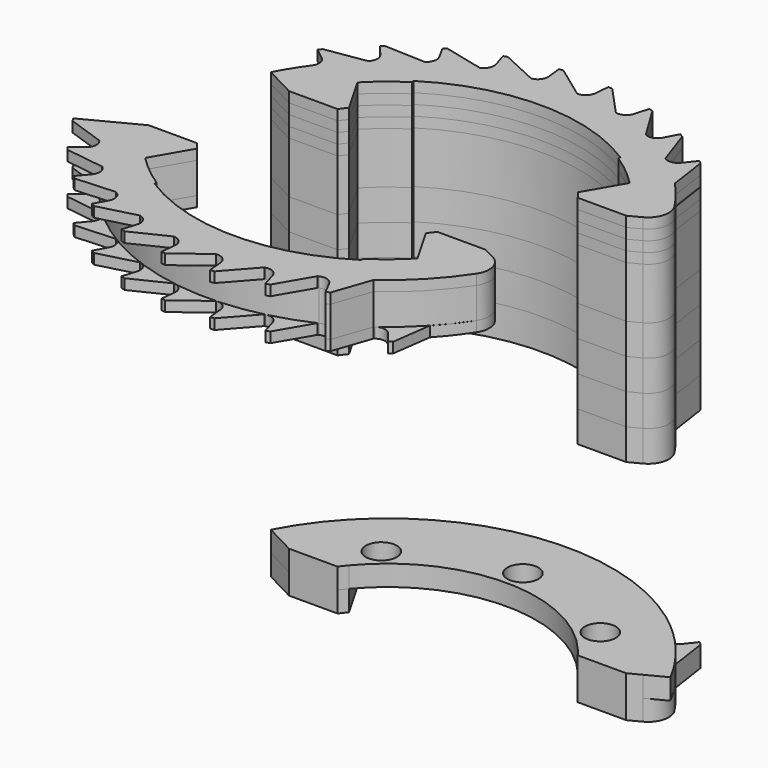
from build123d import *

# Parameters (mm, degrees)
F1_DEPTH  = 1.5
F5_DEPTH  = 0.5
F7_DEPTH  = 0.5
F9_DEPTH  = 0.5
F11_DEPTH = 0.5
F13_DEPTH = 0.5
F15_DEPTH = 0.5
F17_DEPTH = 2.5
F19_DEPTH = 1.5
F21_DEPTH = 1.5
F23_DEPTH = 1.5
F25_DEPTH = 1.5
F28_DEPTH = 1
F29_R     = 0.75
F30_DEPTH = 1


# Not quite as in the source:
# - ends of sketch curves that miss each other by under 0.0002 mm in the source are joined


with BuildPart() as f1:
    # F0 (on Top) → F1 (new body)
    with BuildSketch(Plane.XY):
        with BuildLine():
            Line((5.7645603868, -10.6404813588), (6.3916897173, -8.8292866392))
            ThreePointArc((6.3916897173, -8.8292866392), (5.5229631985, -9.3971739107), (4.6041631591, -9.8798624284))
            ThreePointArc((4.6041631591, -9.8798624284), (4.9761399678, -9.8596213915), (5.2588687206, -10.1021928204))
            Line((5.2588687206, -10.1021928204), (5.5871582201, -10.7328310815))
            Line((5.5871582201, -10.7328310815), (5.7645603868, -10.6404813588))
        make_face()
        with BuildLine():
            ThreePointArc((4.6041631591, -9.8798624284), (5.5229631985, -9.3971739107), (6.3916897173, -8.8292866392))
            ThreePointArc((6.3916897173, -8.8292866392), (7.8806152456, -7.5303322205), (9.110578105, -5.9839256841))
            ThreePointArc((9.110578105, -5.9839256841), (9.2424485693, -5.182849851), (8.7364938645, -4.5479308432))
            Line((8.7364938645, -4.5479308432), (8.1604996652, -4.2480872418))
            Line((8.1604996652, -4.2480872418), (5.813239612, -4.2480872418))
            ThreePointArc((5.813239612, -4.2480872418), (5.6789568424, -4.4259969704), (5.5392313301, -4.5996647999))
            Line((5.5392313301, -4.5996647999), (6.59, -6.4196495231))
            ThreePointArc((6.59, -6.4196495231), (5.8315097631, -7.1157215996), (5, -7.7226938305))
            Line((5, -7.7226938305), (5, -7.841555968))
            ThreePointArc((5, -7.841555968), (0, -9.3), (-5, -7.841555968))
            Line((-5, -7.841555968), (-5, -7.7226938305))
            ThreePointArc((-5, -7.7226938305), (-5.8315097631, -7.1157215996), (-6.59, -6.4196495231))
            Line((-6.59, -6.4196495231), (-5.5392313301, -4.5996647999))
            ThreePointArc((-5.5392313301, -4.5996647999), (-5.6789568424, -4.4259969704), (-5.813239612, -4.2480872418))
            Line((-5.813239612, -4.2480872418), (-8.1604996652, -4.2480872418))
            Line((-8.1604996652, -4.2480872418), (-9.6684180816, -5.0330598843))
            ThreePointArc((-9.6684180816, -5.0330598843), (-3.5049312697, -10.3211170323), (4.6041631591, -9.8798624284))
        make_face()
    extrude(amount=F1_DEPTH)


with BuildPart() as f2_1:
    # F2: copy of F1
    add(f1.part.moved(Location((0, 0, 0.5))))


with BuildPart() as f5:
    # F4 (on face) → F5 (new body)
    with BuildSketch(Plane.XY.offset(1.5)):
        with BuildLine():
            Line((5.7645603868, -10.6404813588), (6.3916897173, -8.8292866392))
            ThreePointArc((6.3916897173, -8.8292866392), (5.5229631985, -9.3971739107), (4.6041631591, -9.8798624284))
            ThreePointArc((4.6041631591, -9.8798624284), (4.9761399678, -9.8596213915), (5.2588687206, -10.1021928204))
            Line((5.2588687206, -10.1021928204), (5.5871582201, -10.7328310815))
            Line((5.5871582201, -10.7328310815), (5.7645603868, -10.6404813588))
        make_face()
        with BuildLine():
            Line((3.5779410407, -11.5606374353), (4.546366818, -9.9065911774))
            ThreePointArc((4.546366818, -9.9065911774), (3.583543325, -10.2940865179), (2.5882299124, -10.5882513155))
            ThreePointArc((2.5882299124, -10.5882513155), (2.9570081214, -10.6409682799), (3.1869809823, -10.9340364101))
            Line((3.1869809823, -10.9340364101), (3.3859310698, -11.6166032381))
            Line((3.3859310698, -11.6166032381), (3.5779410407, -11.5606374353))
        make_face()
        with BuildLine():
            Line((1.2538234269, -12.0365246984), (2.5263295915, -10.6031909723))
            ThreePointArc((2.5263295915, -10.6031909723), (1.5064098912, -10.7954031532), (0.4728324416, -10.8897396425))
            ThreePointArc((0.4728324416, -10.8897396425), (0.8242401112, -11.0133887247), (0.9926193522, -11.3456911126))
            Line((0.9926193522, -11.3456911126), (1.0545844872, -12.0539558469))
            Line((1.0545844872, -12.0539558469), (1.2538234269, -12.0365246984))
        make_face()
        with BuildLine():
            Line((-1.1184779181, -12.0498550675), (0.4092069356, -10.8923160845))
            ThreePointArc((0.4092069356, -10.8923160845), (-0.6286140299, -10.8818584994), (-1.6607357147, -10.7727413821))
            ThreePointArc((-1.6607357147, -10.7727413821), (-1.3402029842, -10.9625708173), (-1.2398880829, -11.3213372683))
            Line((-1.2398880829, -11.3213372683), (-1.3172891857, -12.0280816925))
            Line((-1.3172891857, -12.0280816925), (-1.1184779181, -12.0498550675))
        make_face()
        with BuildLine():
            Line((-3.4477967839, -11.600116264), (-1.7236413133, -10.762855598))
            ThreePointArc((-1.7236413133, -10.762855598), (-2.7394806663, -10.5501301262), (-3.7304827288, -10.2417527118))
            ThreePointArc((-3.7304827288, -10.2417527118), (-3.4531428306, -10.4904674612), (-3.4247473144, -10.8619107818))
            Line((-3.4247473144, -10.8619107818), (-3.638540174, -11.5399751041))
            Line((-3.638540174, -11.5399751041), (-3.4477967839, -11.600116264))
        make_face()
        with BuildLine():
            Line((-5.6446187528, -10.7045914978), (-3.7902509932, -10.2197846068))
            ThreePointArc((-3.7902509932, -10.2197846068), (-4.7450705971, -9.8129661687), (-5.6568693838, -9.3171792284))
            ThreePointArc((-5.6568693838, -9.3171792284), (-5.4333803345, -9.6152213237), (-5.4779954272, -9.9850671555))
            Line((-5.4779954272, -9.9850671555), (-5.8199641039, -10.6083937441))
            Line((-5.8199641039, -10.6083937441), (-5.6446187528, -10.7045914978))
        make_face()
        with BuildLine():
            Line((-7.6245211886, -9.3976952837), (-5.711203453, -9.2839730244))
            ThreePointArc((-5.711203453, -9.2839730244), (-6.5683101259, -8.6986954246), (-7.3658657208, -8.0345517724))
            ThreePointArc((-7.3658657208, -8.0345517724), (-7.2048160792, -8.3704676231), (-7.3207272478, -8.724502998))
            Line((-7.3207272478, -8.724502998), (-7.7777300772, -9.2691377617))
            Line((-7.7777300772, -9.2691377617), (-7.6245211886, -9.3976952837))
        make_face()
        with BuildLine():
            Line((-9.311417551, -7.72965091), (-7.4126775671, -7.9913835652))
            ThreePointArc((-7.4126775671, -7.9913835652), (-8.1391331801, -7.2501386936), (-8.7917959689, -6.4431609976))
            ThreePointArc((-8.7917959689, -6.4431609976), (-8.6993747825, -6.8040415458), (-8.8821276259, -7.1286610831))
            Line((-8.8821276259, -7.1286610831), (-9.4366022454, -7.5736740134))
            Line((-9.4366022454, -7.5736740134), (-9.311417551, -7.72965091))
        make_face()
        with BuildLine():
            ThreePointArc((-8.8292866392, -6.3916897173), (-9.2737661573, -5.7277623256), (-9.6684180816, -5.0330598843))
            Line((-9.6684180816, -5.0330598843), (-10.1021928204, -5.2588687206))
            Line((-10.1021928204, -5.2588687206), (-10.7328310815, -5.5871582201))
            Line((-10.7328310815, -5.5871582201), (-10.6404813588, -5.7645603868))
            Line((-10.6404813588, -5.7645603868), (-8.8292866392, -6.3916897173))
        make_face()
        with BuildLine():
            ThreePointArc((4.6041631591, -9.8798624284), (5.5229631985, -9.3971739107), (6.3916897173, -8.8292866392))
            ThreePointArc((6.3916897173, -8.8292866392), (7.8806152456, -7.5303322205), (9.110578105, -5.9839256841))
            ThreePointArc((9.110578105, -5.9839256841), (9.2424485693, -5.182849851), (8.7364938645, -4.5479308432))
            Line((8.7364938645, -4.5479308432), (8.1604996652, -4.2480872418))
            Line((8.1604996652, -4.2480872418), (5.813239612, -4.2480872418))
            ThreePointArc((5.813239612, -4.2480872418), (5.6789568424, -4.4259969704), (5.5392313301, -4.5996647999))
            Line((5.5392313301, -4.5996647999), (6.59, -6.4196495231))
            ThreePointArc((6.59, -6.4196495231), (5.8315097631, -7.1157215996), (5, -7.7226938305))
            Line((5, -7.7226938305), (5, -7.841555968))
            ThreePointArc((5, -7.841555968), (0, -9.3), (-5, -7.841555968))
            Line((-5, -7.841555968), (-5, -7.7226938305))
            ThreePointArc((-5, -7.7226938305), (-5.8315097631, -7.1157215996), (-6.59, -6.4196495231))
            Line((-6.59, -6.4196495231), (-5.5392313301, -4.5996647999))
            ThreePointArc((-5.5392313301, -4.5996647999), (-5.6789568424, -4.4259969704), (-5.813239612, -4.2480872418))
            Line((-5.813239612, -4.2480872418), (-8.1604996652, -4.2480872418))
            Line((-8.1604996652, -4.2480872418), (-9.6684180816, -5.0330598843))
            ThreePointArc((-9.6684180816, -5.0330598843), (-9.2737661573, -5.7277623256), (-8.8292866392, -6.3916897173))
            ThreePointArc((-8.8292866392, -6.3916897173), (-8.810578891, -6.417452735), (-8.7917959689, -6.4431609976))
            ThreePointArc((-8.7917959689, -6.4431609976), (-8.1391331801, -7.2501386936), (-7.4126775671, -7.9913835652))
            ThreePointArc((-7.4126775671, -7.9913835652), (-7.3893031675, -8.0130018532), (-7.3658657208, -8.0345517724))
            ThreePointArc((-7.3658657208, -8.0345517724), (-6.5683101259, -8.6986954246), (-5.711203453, -9.2839730244))
            ThreePointArc((-5.711203453, -9.2839730244), (-5.6840606672, -9.3006158039), (-5.6568693838, -9.3171792284))
            ThreePointArc((-5.6568693838, -9.3171792284), (-4.7450705971, -9.8129661687), (-3.7902509932, -10.2197846068))
            ThreePointArc((-3.7902509932, -10.2197846068), (-3.7603829032, -10.230812305), (-3.7304827288, -10.2417527118))
            ThreePointArc((-3.7304827288, -10.2417527118), (-2.7394806663, -10.5501301262), (-1.7236413133, -10.762855598))
            ThreePointArc((-1.7236413133, -10.762855598), (-1.6921957331, -10.7678444269), (-1.6607357147, -10.7727413821))
            ThreePointArc((-1.6607357147, -10.7727413821), (-0.6286140299, -10.8818584994), (0.4092069356, -10.8923160845))
            ThreePointArc((0.4092069356, -10.8923160845), (0.4410215701, -10.891074326), (0.4728324416, -10.8897396425))
            ThreePointArc((0.4728324416, -10.8897396425), (1.5064098912, -10.7954031532), (2.5263295915, -10.6031909723))
            ThreePointArc((2.5263295915, -10.6031909723), (2.5572906616, -10.5957663466), (2.5882299124, -10.5882513155))
            ThreePointArc((2.5882299124, -10.5882513155), (3.583543325, -10.2940865179), (4.546366818, -9.9065911774))
            ThreePointArc((4.546366818, -9.9065911774), (4.5752845072, -9.8932690087), (4.6041631591, -9.8798624284))
        make_face()
    extrude(amount=F5_DEPTH)


with BuildPart() as f7:
    # F6 (on Top) → F7 (new body)
    with BuildSketch(Plane.XY):
        with BuildLine():
            Line((5.7645603868, -10.6404813588), (6.3916897173, -8.8292866392))
            ThreePointArc((6.3916897173, -8.8292866392), (5.5229631985, -9.3971739107), (4.6041631591, -9.8798624284))
            ThreePointArc((4.6041631591, -9.8798624284), (4.9761399678, -9.8596213915), (5.2588687206, -10.1021928204))
            Line((5.2588687206, -10.1021928204), (5.5871582201, -10.7328310815))
            Line((5.5871582201, -10.7328310815), (5.7645603868, -10.6404813588))
        make_face()
        with BuildLine():
            ThreePointArc((4.6041631591, -9.8798624284), (5.5229631985, -9.3971739107), (6.3916897173, -8.8292866392))
            ThreePointArc((6.3916897173, -8.8292866392), (6.417452735, -8.810578891), (6.4431609976, -8.7917959689))
            ThreePointArc((6.4431609976, -8.7917959689), (7.2501386936, -8.1391331801), (7.9913835652, -7.4126775671))
            ThreePointArc((7.9913835652, -7.4126775671), (8.5807695592, -6.7216362422), (9.110578105, -5.9839256841))
            ThreePointArc((9.110578105, -5.9839256841), (9.2424485693, -5.182849851), (8.7364938645, -4.5479308432))
            Line((8.7364938645, -4.5479308432), (8.1604996652, -4.2480872418))
            Line((8.1604996652, -4.2480872418), (5.813239612, -4.2480872418))
            ThreePointArc((5.813239612, -4.2480872418), (5.6789568424, -4.4259969704), (5.5392313301, -4.5996647999))
            Line((5.5392313301, -4.5996647999), (6.59, -6.4196495231))
            ThreePointArc((6.59, -6.4196495231), (5.8315097631, -7.1157215996), (5, -7.7226938305))
            Line((5, -7.7226938305), (5, -7.841555968))
            ThreePointArc((5, -7.841555968), (0, -9.3), (-5, -7.841555968))
            Line((-5, -7.841555968), (-5, -7.7226938305))
            ThreePointArc((-5, -7.7226938305), (-5.8315097631, -7.1157215996), (-6.59, -6.4196495231))
            Line((-6.59, -6.4196495231), (-5.5392313301, -4.5996647999))
            ThreePointArc((-5.5392313301, -4.5996647999), (-5.6789568424, -4.4259969704), (-5.813239612, -4.2480872418))
            Line((-5.813239612, -4.2480872418), (-8.1604996652, -4.2480872418))
            Line((-8.1604996652, -4.2480872418), (-9.6684180816, -5.0330598843))
            ThreePointArc((-9.6684180816, -5.0330598843), (-9.2737661573, -5.7277623256), (-8.8292866392, -6.3916897173))
            ThreePointArc((-8.8292866392, -6.3916897173), (-8.810578891, -6.417452735), (-8.7917959689, -6.4431609976))
            ThreePointArc((-8.7917959689, -6.4431609976), (-8.1391331801, -7.2501386936), (-7.4126775671, -7.9913835652))
            ThreePointArc((-7.4126775671, -7.9913835652), (-7.3893031675, -8.0130018532), (-7.3658657208, -8.0345517724))
            ThreePointArc((-7.3658657208, -8.0345517724), (-6.5683101259, -8.6986954246), (-5.711203453, -9.2839730244))
            ThreePointArc((-5.711203453, -9.2839730244), (-5.6840606672, -9.3006158039), (-5.6568693838, -9.3171792284))
            ThreePointArc((-5.6568693838, -9.3171792284), (-4.7450705971, -9.8129661687), (-3.7902509932, -10.2197846068))
            ThreePointArc((-3.7902509932, -10.2197846068), (-3.7603829032, -10.230812305), (-3.7304827288, -10.2417527118))
            ThreePointArc((-3.7304827288, -10.2417527118), (-2.7394806663, -10.5501301262), (-1.7236413133, -10.762855598))
            ThreePointArc((-1.7236413133, -10.762855598), (-1.6921957331, -10.7678444269), (-1.6607357147, -10.7727413821))
            ThreePointArc((-1.6607357147, -10.7727413821), (-0.6286140299, -10.8818584994), (0.4092069356, -10.8923160845))
            ThreePointArc((0.4092069356, -10.8923160845), (0.4410215701, -10.891074326), (0.4728324416, -10.8897396425))
            ThreePointArc((0.4728324416, -10.8897396425), (1.5064098912, -10.7954031532), (2.5263295915, -10.6031909723))
            ThreePointArc((2.5263295915, -10.6031909723), (2.5572906616, -10.5957663466), (2.5882299124, -10.5882513155))
            ThreePointArc((2.5882299124, -10.5882513155), (3.583543325, -10.2940865179), (4.546366818, -9.9065911774))
            ThreePointArc((4.546366818, -9.9065911774), (4.5752845072, -9.8932690087), (4.6041631591, -9.8798624284))
        make_face()
        with BuildLine():
            ThreePointArc((7.9913835652, -7.4126775671), (7.2501386936, -8.1391331801), (6.4431609976, -8.7917959689))
            ThreePointArc((6.4431609976, -8.7917959689), (6.8040415458, -8.6993747825), (7.1286610831, -8.8821276259))
            Line((7.1286610831, -8.8821276259), (7.5736740134, -9.4366022454))
            Line((7.5736740134, -9.4366022454), (7.72965091, -9.311417551))
            Line((7.72965091, -9.311417551), (7.9913835652, -7.4126775671))
        make_face()
        with BuildLine():
            Line((3.5779410407, -11.5606374353), (4.546366818, -9.9065911774))
            ThreePointArc((4.546366818, -9.9065911774), (3.583543325, -10.2940865179), (2.5882299124, -10.5882513155))
            ThreePointArc((2.5882299124, -10.5882513155), (2.9570081214, -10.6409682799), (3.1869809823, -10.9340364101))
            Line((3.1869809823, -10.9340364101), (3.3859310698, -11.6166032381))
            Line((3.3859310698, -11.6166032381), (3.5779410407, -11.5606374353))
        make_face()
        with BuildLine():
            Line((1.2538234269, -12.0365246984), (2.5263295915, -10.6031909723))
            ThreePointArc((2.5263295915, -10.6031909723), (1.5064098912, -10.7954031532), (0.4728324416, -10.8897396425))
            ThreePointArc((0.4728324416, -10.8897396425), (0.8242401112, -11.0133887247), (0.9926193522, -11.3456911126))
            Line((0.9926193522, -11.3456911126), (1.0545844872, -12.0539558469))
            Line((1.0545844872, -12.0539558469), (1.2538234269, -12.0365246984))
        make_face()
        with BuildLine():
            Line((-1.1184779181, -12.0498550675), (0.4092069356, -10.8923160845))
            ThreePointArc((0.4092069356, -10.8923160845), (-0.6286140299, -10.8818584994), (-1.6607357147, -10.7727413821))
            ThreePointArc((-1.6607357147, -10.7727413821), (-1.3402029842, -10.9625708173), (-1.2398880829, -11.3213372683))
            Line((-1.2398880829, -11.3213372683), (-1.3172891857, -12.0280816925))
            Line((-1.3172891857, -12.0280816925), (-1.1184779181, -12.0498550675))
        make_face()
        with BuildLine():
            Line((-3.4477967839, -11.600116264), (-1.7236413133, -10.762855598))
            ThreePointArc((-1.7236413133, -10.762855598), (-2.7394806663, -10.5501301262), (-3.7304827288, -10.2417527118))
            ThreePointArc((-3.7304827288, -10.2417527118), (-3.4531428306, -10.4904674612), (-3.4247473144, -10.8619107818))
            Line((-3.4247473144, -10.8619107818), (-3.638540174, -11.5399751041))
            Line((-3.638540174, -11.5399751041), (-3.4477967839, -11.600116264))
        make_face()
        with BuildLine():
            Line((-5.6446187528, -10.7045914978), (-3.7902509932, -10.2197846068))
            ThreePointArc((-3.7902509932, -10.2197846068), (-4.7450705971, -9.8129661687), (-5.6568693838, -9.3171792284))
            ThreePointArc((-5.6568693838, -9.3171792284), (-5.4333803345, -9.6152213237), (-5.4779954272, -9.9850671555))
            Line((-5.4779954272, -9.9850671555), (-5.8199641039, -10.6083937441))
            Line((-5.8199641039, -10.6083937441), (-5.6446187528, -10.7045914978))
        make_face()
        with BuildLine():
            Line((-7.6245211886, -9.3976952837), (-5.711203453, -9.2839730244))
            ThreePointArc((-5.711203453, -9.2839730244), (-6.5683101259, -8.6986954246), (-7.3658657208, -8.0345517724))
            ThreePointArc((-7.3658657208, -8.0345517724), (-7.2048160792, -8.3704676231), (-7.3207272478, -8.724502998))
            Line((-7.3207272478, -8.724502998), (-7.7777300772, -9.2691377617))
            Line((-7.7777300772, -9.2691377617), (-7.6245211886, -9.3976952837))
        make_face()
        with BuildLine():
            Line((-9.311417551, -7.72965091), (-7.4126775671, -7.9913835652))
            ThreePointArc((-7.4126775671, -7.9913835652), (-8.1391331801, -7.2501386936), (-8.7917959689, -6.4431609976))
            ThreePointArc((-8.7917959689, -6.4431609976), (-8.6993747825, -6.8040415458), (-8.8821276259, -7.1286610831))
            Line((-8.8821276259, -7.1286610831), (-9.4366022454, -7.5736740134))
            Line((-9.4366022454, -7.5736740134), (-9.311417551, -7.72965091))
        make_face()
        with BuildLine():
            Line((-10.6404813588, -5.7645603868), (-8.8292866392, -6.3916897173))
            ThreePointArc((-8.8292866392, -6.3916897173), (-9.2737661573, -5.7277623256), (-9.6684180816, -5.0330598843))
            Line((-9.6684180816, -5.0330598843), (-10.1021928204, -5.2588687206))
            Line((-10.1021928204, -5.2588687206), (-10.7328310815, -5.5871582201))
            Line((-10.7328310815, -5.5871582201), (-10.6404813588, -5.7645603868))
        make_face()
    extrude(amount=-F7_DEPTH)


with BuildPart() as f9:
    # F8 (on face) → F9 (new body)
    with BuildSketch(Plane(origin=(0, 0, -0.5), x_dir=(1, 0, 0), z_dir=(0, 0, -1))):
        with BuildLine():
            Line((5.7645603868, -10.6404813588), (6.3916897173, -8.8292866392))
            ThreePointArc((6.3916897173, -8.8292866392), (5.5229631985, -9.3971739107), (4.6041631591, -9.8798624284))
            ThreePointArc((4.6041631591, -9.8798624284), (4.9761399678, -9.8596213915), (5.2588687206, -10.1021928204))
            Line((5.2588687206, -10.1021928204), (5.5871582201, -10.7328310815))
            Line((5.5871582201, -10.7328310815), (5.7645603868, -10.6404813588))
        make_face()
        with BuildLine():
            Line((3.5779410407, -11.5606374353), (4.6041631591, -9.8798624284))
            ThreePointArc((4.6041631591, -9.8798624284), (3.613596993, -10.2835750968), (2.5882299124, -10.5882513155))
            ThreePointArc((2.5882299124, -10.5882513155), (2.9570081214, -10.6409682799), (3.1869809823, -10.9340364101))
            Line((3.1869809823, -10.9340364101), (3.3859310698, -11.6166032381))
            Line((3.3859310698, -11.6166032381), (3.5779410407, -11.5606374353))
        make_face()
        with BuildLine():
            Line((1.2538234269, -12.0365246984), (2.5882299124, -10.5882513155))
            ThreePointArc((2.5882299124, -10.5882513155), (1.5379367629, -10.7909568859), (0.4728324416, -10.8897396425))
            ThreePointArc((0.4728324416, -10.8897396425), (0.8242401112, -11.0133887247), (0.9926193522, -11.3456911126))
            Line((0.9926193522, -11.3456911126), (1.0545844872, -12.0539558469))
            Line((1.0545844872, -12.0539558469), (1.2538234269, -12.0365246984))
        make_face()
        with BuildLine():
            Line((-1.1184779181, -12.0498550675), (0.4728324416, -10.8897396425))
            ThreePointArc((0.4728324416, -10.8897396425), (-0.5968255145, -10.8836482535), (-1.6607357147, -10.7727413821))
            ThreePointArc((-1.6607357147, -10.7727413821), (-1.3402029842, -10.9625708173), (-1.2398880829, -11.3213372683))
            Line((-1.2398880829, -11.3213372683), (-1.3172891857, -12.0280816925))
            Line((-1.3172891857, -12.0280816925), (-1.1184779181, -12.0498550675))
        make_face()
        with BuildLine():
            Line((-3.4477967839, -11.600116264), (-1.6607357147, -10.7727413821))
            ThreePointArc((-1.6607357147, -10.7727413821), (-2.7086521221, -10.5580871223), (-3.7304827288, -10.2417527118))
            ThreePointArc((-3.7304827288, -10.2417527118), (-3.4531428306, -10.4904674612), (-3.4247473144, -10.8619107818))
            Line((-3.4247473144, -10.8619107818), (-3.638540174, -11.5399751041))
            Line((-3.638540174, -11.5399751041), (-3.4477967839, -11.600116264))
        make_face()
        with BuildLine():
            Line((-5.6446187528, -10.7045914978), (-3.7304827288, -10.2417527118))
            ThreePointArc((-3.7304827288, -10.2417527118), (-4.7163867476, -9.826784624), (-5.6568693838, -9.3171792284))
            ThreePointArc((-5.6568693838, -9.3171792284), (-5.4333803345, -9.6152213237), (-5.4779954272, -9.9850671555))
            Line((-5.4779954272, -9.9850671555), (-5.8199641039, -10.6083937441))
            Line((-5.8199641039, -10.6083937441), (-5.6446187528, -10.7045914978))
        make_face()
        with BuildLine():
            Line((-7.6245211886, -9.3976952837), (-5.6568693838, -9.3171792284))
            ThreePointArc((-5.6568693838, -9.3171792284), (-6.5428732754, -8.7178443036), (-7.3658657208, -8.0345517724))
            ThreePointArc((-7.3658657208, -8.0345517724), (-7.2048160792, -8.3704676231), (-7.3207272478, -8.724502998))
            Line((-7.3207272478, -8.724502998), (-7.7777300772, -9.2691377617))
            Line((-7.7777300772, -9.2691377617), (-7.6245211886, -9.3976952837))
        make_face()
        with BuildLine():
            Line((-9.311417551, -7.72965091), (-7.3658657208, -8.0345517724))
            ThreePointArc((-7.3658657208, -8.0345517724), (-8.1179208526, -7.2738821156), (-8.7917959689, -6.4431609976))
            ThreePointArc((-8.7917959689, -6.4431609976), (-8.6993747825, -6.8040415458), (-8.8821276259, -7.1286610831))
            Line((-8.8821276259, -7.1286610831), (-9.4366022454, -7.5736740134))
            Line((-9.4366022454, -7.5736740134), (-9.311417551, -7.72965091))
        make_face()
        with BuildLine():
            ThreePointArc((7.9451671881, -7.4621925969), (7.2009445916, -8.1826888606), (6.3916897173, -8.8292866392))
            ThreePointArc((6.3916897173, -8.8292866392), (6.7529700924, -8.7384409661), (7.0767891323, -8.9226084852))
            Line((7.0767891323, -8.9226084852), (7.5193784822, -9.4790195556))
            Line((7.5193784822, -9.4790195556), (7.6759001136, -9.3545166283))
            Line((7.6759001136, -9.3545166283), (7.9451671881, -7.4621925969))
        make_face()
        with BuildLine():
            ThreePointArc((4.6041631591, -9.8798624284), (5.5229631985, -9.3971739107), (6.3916897173, -8.8292866392))
            ThreePointArc((6.3916897173, -8.8292866392), (7.2009445916, -8.1826888606), (7.9451671881, -7.4621925969))
            ThreePointArc((7.9451671881, -7.4621925969), (8.5598440489, -6.7482642108), (9.110578105, -5.9839256841))
            ThreePointArc((9.110578105, -5.9839256841), (9.2424485693, -5.182849851), (8.7364938645, -4.5479308432))
            Line((8.7364938645, -4.5479308432), (8.1604996652, -4.2480872418))
            Line((8.1604996652, -4.2480872418), (5.813239612, -4.2480872418))
            ThreePointArc((5.813239612, -4.2480872418), (5.6789568424, -4.4259969704), (5.5392313301, -4.5996647999))
            Line((5.5392313301, -4.5996647999), (6.59, -6.4196495231))
            ThreePointArc((6.59, -6.4196495231), (5.8315097631, -7.1157215996), (5, -7.7226938305))
            Line((5, -7.7226938305), (5, -7.841555968))
            ThreePointArc((5, -7.841555968), (0, -9.3), (-5, -7.841555968))
            Line((-5, -7.841555968), (-5, -7.7226938305))
            ThreePointArc((-5, -7.7226938305), (-5.8315097631, -7.1157215996), (-6.59, -6.4196495231))
            Line((-6.59, -6.4196495231), (-5.5392313301, -4.5996647999))
            ThreePointArc((-5.5392313301, -4.5996647999), (-5.6789568424, -4.4259969704), (-5.813239612, -4.2480872418))
            Line((-5.813239612, -4.2480872418), (-8.1604996652, -4.2480872418))
            Line((-8.1604996652, -4.2480872418), (-9.6684180816, -5.0330598843))
            ThreePointArc((-9.6684180816, -5.0330598843), (-9.2569958402, -5.7548264974), (-8.7917959689, -6.4431609976))
            ThreePointArc((-8.7917959689, -6.4431609976), (-8.1179208526, -7.2738821156), (-7.3658657208, -8.0345517724))
            ThreePointArc((-7.3658657208, -8.0345517724), (-6.5428732754, -8.7178443036), (-5.6568693838, -9.3171792284))
            ThreePointArc((-5.6568693838, -9.3171792284), (-4.7163867476, -9.826784624), (-3.7304827288, -10.2417527118))
            ThreePointArc((-3.7304827288, -10.2417527118), (-2.7086521221, -10.5580871223), (-1.6607357147, -10.7727413821))
            ThreePointArc((-1.6607357147, -10.7727413821), (-0.5968255145, -10.8836482535), (0.4728324416, -10.8897396425))
            ThreePointArc((0.4728324416, -10.8897396425), (1.5379367629, -10.7909568859), (2.5882299124, -10.5882513155))
            ThreePointArc((2.5882299124, -10.5882513155), (3.613596993, -10.2835750968), (4.6041631591, -9.8798624284))
        make_face()
    extrude(amount=-F9_DEPTH)


with BuildPart() as f11:
    # F10 (on face) → F11 (new body)
    with BuildSketch(Plane(origin=(0, 0, -0.5), x_dir=(1, 0, 0), z_dir=(0, 0, -1))):
        with BuildLine():
            Line((5.7645603868, -10.6404813588), (6.3916897173, -8.8292866392))
            ThreePointArc((6.3916897173, -8.8292866392), (5.5229631985, -9.3971739107), (4.6041631591, -9.8798624284))
            ThreePointArc((4.6041631591, -9.8798624284), (4.9761399678, -9.8596213915), (5.2588687206, -10.1021928204))
            Line((5.2588687206, -10.1021928204), (5.5871582201, -10.7328310815))
            Line((5.5871582201, -10.7328310815), (5.7645603868, -10.6404813588))
        make_face()
        with BuildLine():
            ThreePointArc((4.6041631591, -9.8798624284), (5.5229631985, -9.3971739107), (6.3916897173, -8.8292866392))
            ThreePointArc((6.3916897173, -8.8292866392), (7.2009445916, -8.1826888606), (7.9451671881, -7.4621925969))
            ThreePointArc((7.9451671881, -7.4621925969), (8.5598440489, -6.7482642108), (9.110578105, -5.9839256841))
            ThreePointArc((9.110578105, -5.9839256841), (9.2424485693, -5.182849851), (8.7364938645, -4.5479308432))
            Line((8.7364938645, -4.5479308432), (8.1604996652, -4.2480872418))
            Line((8.1604996652, -4.2480872418), (5.813239612, -4.2480872418))
            ThreePointArc((5.813239612, -4.2480872418), (5.6789568424, -4.4259969704), (5.5392313301, -4.5996647999))
            Line((5.5392313301, -4.5996647999), (6.59, -6.4196495231))
            ThreePointArc((6.59, -6.4196495231), (5.8315097631, -7.1157215996), (5, -7.7226938305))
            Line((5, -7.7226938305), (5, -7.841555968))
            ThreePointArc((5, -7.841555968), (0, -9.3), (-5, -7.841555968))
            Line((-5, -7.841555968), (-5, -7.7226938305))
            ThreePointArc((-5, -7.7226938305), (-5.8315097631, -7.1157215996), (-6.59, -6.4196495231))
            Line((-6.59, -6.4196495231), (-5.5392313301, -4.5996647999))
            ThreePointArc((-5.5392313301, -4.5996647999), (-5.6789568424, -4.4259969704), (-5.813239612, -4.2480872418))
            Line((-5.813239612, -4.2480872418), (-8.1604996652, -4.2480872418))
            Line((-8.1604996652, -4.2480872418), (-9.6684180816, -5.0330598843))
            ThreePointArc((-9.6684180816, -5.0330598843), (-8.6483492387, -6.6344596951), (-7.3658657208, -8.0345517724))
            ThreePointArc((-7.3658657208, -8.0345517724), (-6.5428732754, -8.7178443036), (-5.6568693838, -9.3171792284))
            ThreePointArc((-5.6568693838, -9.3171792284), (-4.7163867476, -9.826784624), (-3.7304827288, -10.2417527118))
            ThreePointArc((-3.7304827288, -10.2417527118), (-2.7086521221, -10.5580871223), (-1.6607357147, -10.7727413821))
            ThreePointArc((-1.6607357147, -10.7727413821), (-0.5968255145, -10.8836482535), (0.4728324416, -10.8897396425))
            ThreePointArc((0.4728324416, -10.8897396425), (1.5379367629, -10.7909568859), (2.5882299124, -10.5882513155))
            ThreePointArc((2.5882299124, -10.5882513155), (3.613596993, -10.2835750968), (4.6041631591, -9.8798624284))
        make_face()
        with BuildLine():
            ThreePointArc((7.9451671881, -7.4621925969), (7.2009445916, -8.1826888606), (6.3916897173, -8.8292866392))
            ThreePointArc((6.3916897173, -8.8292866392), (6.7529700924, -8.7384409661), (7.0767891323, -8.9226084852))
            Line((7.0767891323, -8.9226084852), (7.5193784822, -9.4790195556))
            Line((7.5193784822, -9.4790195556), (7.6759001136, -9.3545166283))
            Line((7.6759001136, -9.3545166283), (7.9451671881, -7.4621925969))
        make_face()
        with BuildLine():
            Line((3.5779410407, -11.5606374353), (4.6041631591, -9.8798624284))
            ThreePointArc((4.6041631591, -9.8798624284), (3.613596993, -10.2835750968), (2.5882299124, -10.5882513155))
            ThreePointArc((2.5882299124, -10.5882513155), (2.9570081214, -10.6409682799), (3.1869809823, -10.9340364101))
            Line((3.1869809823, -10.9340364101), (3.3859310698, -11.6166032381))
            Line((3.3859310698, -11.6166032381), (3.5779410407, -11.5606374353))
        make_face()
        with BuildLine():
            Line((1.2538234269, -12.0365246984), (2.5882299124, -10.5882513155))
            ThreePointArc((2.5882299124, -10.5882513155), (1.5379367629, -10.7909568859), (0.4728324416, -10.8897396425))
            ThreePointArc((0.4728324416, -10.8897396425), (0.8242401112, -11.0133887247), (0.9926193522, -11.3456911126))
            Line((0.9926193522, -11.3456911126), (1.0545844872, -12.0539558469))
            Line((1.0545844872, -12.0539558469), (1.2538234269, -12.0365246984))
        make_face()
        with BuildLine():
            Line((-1.1184779181, -12.0498550675), (0.4728324416, -10.8897396425))
            ThreePointArc((0.4728324416, -10.8897396425), (-0.5968255145, -10.8836482535), (-1.6607357147, -10.7727413821))
            ThreePointArc((-1.6607357147, -10.7727413821), (-1.3402029842, -10.9625708173), (-1.2398880829, -11.3213372683))
            Line((-1.2398880829, -11.3213372683), (-1.3172891857, -12.0280816925))
            Line((-1.3172891857, -12.0280816925), (-1.1184779181, -12.0498550675))
        make_face()
        with BuildLine():
            Line((-3.4477967839, -11.600116264), (-1.6607357147, -10.7727413821))
            ThreePointArc((-1.6607357147, -10.7727413821), (-2.7086521221, -10.5580871223), (-3.7304827288, -10.2417527118))
            ThreePointArc((-3.7304827288, -10.2417527118), (-3.4531428306, -10.4904674612), (-3.4247473144, -10.8619107818))
            Line((-3.4247473144, -10.8619107818), (-3.638540174, -11.5399751041))
            Line((-3.638540174, -11.5399751041), (-3.4477967839, -11.600116264))
        make_face()
        with BuildLine():
            Line((-5.6446187528, -10.7045914978), (-3.7304827288, -10.2417527118))
            ThreePointArc((-3.7304827288, -10.2417527118), (-4.7163867476, -9.826784624), (-5.6568693838, -9.3171792284))
            ThreePointArc((-5.6568693838, -9.3171792284), (-5.4333803345, -9.6152213237), (-5.4779954272, -9.9850671555))
            Line((-5.4779954272, -9.9850671555), (-5.8199641039, -10.6083937441))
            Line((-5.8199641039, -10.6083937441), (-5.6446187528, -10.7045914978))
        make_face()
        with BuildLine():
            Line((-7.6245211886, -9.3976952837), (-5.6568693838, -9.3171792284))
            ThreePointArc((-5.6568693838, -9.3171792284), (-6.5428732754, -8.7178443036), (-7.3658657208, -8.0345517724))
            ThreePointArc((-7.3658657208, -8.0345517724), (-7.2048160792, -8.3704676231), (-7.3207272478, -8.724502998))
            Line((-7.3207272478, -8.724502998), (-7.7777300772, -9.2691377617))
            Line((-7.7777300772, -9.2691377617), (-7.6245211886, -9.3976952837))
        make_face()
    extrude(amount=F11_DEPTH)


with BuildPart() as f13:
    # F12 (on face) → F13 (new body)
    with BuildSketch(Plane(origin=(0, 0, -1), x_dir=(1, 0, 0), z_dir=(0, 0, -1))):
        with BuildLine():
            ThreePointArc((9.1100288204, -5.984761891), (9.1103035022, -5.9843437482), (9.1105781649, -5.9839255929))
            ThreePointArc((9.1105781649, -5.9839255929), (9.2424486233, -5.1828497668), (8.7364939254, -4.5479307637))
            Line((8.7364939254, -4.5479307637), (8.160499713, -4.2480871501))
            Line((8.160499713, -4.2480871501), (5.813239679, -4.2480871501))
            ThreePointArc((5.813239679, -4.2480871501), (5.6789569122, -4.4259968809), (5.5392314026, -4.5996647126))
            Line((5.5392314026, -4.5996647126), (6.59, -6.4196495231))
            ThreePointArc((6.59, -6.4196495231), (5.8315097631, -7.1157215996), (5, -7.7226938305))
            Line((5, -7.7226938305), (5, -7.841555968))
            ThreePointArc((5, -7.841555968), (0, -9.3), (-5, -7.841555968))
            Line((-5, -7.841555968), (-5, -7.7226938305))
            ThreePointArc((-5, -7.7226938305), (-5.8315097631, -7.1157215996), (-6.59, -6.4196495231))
            Line((-6.59, -6.4196495231), (-5.5392312576, -4.5996648872))
            ThreePointArc((-5.5392312576, -4.5996648872), (-5.6789567726, -4.42599706), (-5.813239545, -4.2480873334))
            Line((-5.813239545, -4.2480873334), (-8.1604996175, -4.2480873334))
            Line((-8.1604996175, -4.2480873334), (-9.6684180251, -5.0330599928))
            ThreePointArc((-9.6684180251, -5.0330599928), (-7.9564141976, -7.4501995353), (-5.6568692166, -9.31717933))
            ThreePointArc((-5.6568692166, -9.31717933), (-4.7163865698, -9.8267847094), (-3.730482542, -10.2417527799))
            ThreePointArc((-3.730482542, -10.2417527799), (-2.7086519295, -10.5580871717), (-1.6607355182, -10.7727414124))
            ThreePointArc((-1.6607355182, -10.7727414124), (-0.596825316, -10.8836482644), (0.4728326403, -10.8897396339))
            ThreePointArc((0.4728326403, -10.8897396339), (1.5379369597, -10.7909568578), (2.5882301055, -10.5882512683))
            ThreePointArc((2.5882301055, -10.5882512683), (3.6135971445, -10.2835750436), (4.6041632701, -9.8798623767))
            ThreePointArc((4.6041632701, -9.8798623767), (5.52990946, -9.3930879568), (6.4047384375, -8.8198257096))
            ThreePointArc((6.4047384375, -8.8198257096), (7.2205951244, -8.1653540064), (7.9699674361, -7.4356989629))
            ThreePointArc((7.9699674361, -7.4356989629), (8.5707568293, -6.734398813), (9.1100288204, -5.984761891))
        make_face()
        with BuildLine():
            Line((7.6889488396, -9.3450556842), (7.9699674361, -7.4356989629))
            ThreePointArc((7.9699674361, -7.4356989629), (7.2205951244, -8.1653540064), (6.4047384375, -8.8198257096))
            ThreePointArc((6.4047384375, -8.8198257096), (6.7660188115, -8.7289800323), (7.0898378536, -8.9131475479))
            Line((7.0898378536, -8.9131475479), (7.5324272097, -9.4695586133))
            Line((7.5324272097, -9.4695586133), (7.6889488396, -9.3450556842))
        make_face()
        with BuildLine():
            Line((5.7645605063, -10.6404812941), (6.4047384375, -8.8198257096))
            ThreePointArc((6.4047384375, -8.8198257096), (5.52990946, -9.3930879568), (4.6041632701, -9.8798623767))
            ThreePointArc((4.6041632701, -9.8798623767), (4.9761400785, -9.8596213357), (5.2588688341, -10.1021927613))
            Line((5.2588688341, -10.1021927613), (5.5871583407, -10.7328310187))
            Line((5.5871583407, -10.7328310187), (5.7645605063, -10.6404812941))
        make_face()
        with BuildLine():
            Line((3.5779411516, -11.5606373836), (4.6041632701, -9.8798623767))
            ThreePointArc((4.6041632701, -9.8798623767), (3.6135971445, -10.2835750436), (2.5882301055, -10.5882512683))
            ThreePointArc((2.5882301024, -10.5882512691), (2.9570083124, -10.6409682268), (3.1869811786, -10.9340363529))
            Line((3.1869811786, -10.9340363529), (3.3859312608, -11.616603163))
            Line((3.3859312608, -11.616603163), (3.5779411516, -11.5606373836))
        make_face()
        with BuildLine():
            Line((1.2538236305, -12.0365246805), (2.588230116, -10.5882512977))
            ThreePointArc((2.5882301055, -10.5882512683), (1.5379369597, -10.7909568578), (0.4728326403, -10.8897396339))
            ThreePointArc((0.4728326371, -10.889739634), (0.8242403089, -11.01338871), (0.9926195559, -11.3456910947))
            Line((0.9926195559, -11.3456910947), (1.0545846909, -12.0539558291))
            Line((1.0545846909, -12.0539558291), (1.2538236305, -12.0365246805))
        make_face()
        with BuildLine():
            Line((-1.1184777149, -12.0498550897), (0.4728326448, -10.8897396648))
            ThreePointArc((0.4728326403, -10.8897396339), (-0.596825316, -10.8836482644), (-1.6607355182, -10.7727414124))
            ThreePointArc((-1.6607355213, -10.7727414119), (-1.3402027875, -10.9625708414), (-1.2398878798, -11.3213372905))
            Line((-1.2398878798, -11.3213372905), (-1.3172889825, -12.0280817147))
            Line((-1.3172889825, -12.0280817147), (-1.1184777149, -12.0498550897))
        make_face()
        with BuildLine():
            Line((-3.4477965889, -11.6001163254), (-1.6607355197, -10.7727414436))
            ThreePointArc((-1.6607355182, -10.7727414124), (-2.7086519295, -10.5580871717), (-3.730482542, -10.2417527799))
            ThreePointArc((-3.730482545, -10.2417527788), (-3.4531426423, -10.4904675232), (-3.4247471195, -10.8619108433))
            Line((-3.4247471195, -10.8619108433), (-3.638539979, -11.5399751655))
            Line((-3.638539979, -11.5399751655), (-3.4477965889, -11.6001163254))
        make_face()
        with BuildLine():
            Line((-5.6446185736, -10.7045915962), (-3.7304825496, -10.2417528101))
            ThreePointArc((-3.730482542, -10.2417527799), (-4.7163865698, -9.8267847094), (-5.6568692166, -9.31717933))
            ThreePointArc((-5.6568692166, -9.31717933), (-5.4333801619, -9.6152214213), (-5.477995248, -9.9850672538))
            Line((-5.477995248, -9.9850672538), (-5.8199639247, -10.6083938424))
            Line((-5.8199639247, -10.6083938424), (-5.6446185736, -10.7045915962))
        make_face()
    extrude(amount=F13_DEPTH)


with BuildPart() as f15:
    # F14 (on face) → F15 (new body)
    with BuildSketch(Plane(origin=(0, 0, -1.5), x_dir=(1, 0, 0), z_dir=(0, 0, -1))):
        with BuildLine():
            Line((7.6889488396, -9.3450556842), (7.9699674361, -7.4356989629))
            ThreePointArc((7.9699674361, -7.4356989629), (7.2205951244, -8.1653540064), (6.4047384375, -8.8198257096))
            ThreePointArc((6.4047384375, -8.8198257096), (6.7660188115, -8.7289800323), (7.0898378536, -8.9131475479))
            Line((7.0898378536, -8.9131475479), (7.5324272097, -9.4695586133))
            Line((7.5324272097, -9.4695586133), (7.6889488396, -9.3450556842))
        make_face()
        with BuildLine():
            Line((5.7645605063, -10.6404812941), (6.4047384375, -8.8198257096))
            ThreePointArc((6.4047384375, -8.8198257096), (5.52990946, -9.3930879568), (4.6041632701, -9.8798623767))
            ThreePointArc((4.6041632701, -9.8798623767), (4.9761400785, -9.8596213357), (5.2588688341, -10.1021927613))
            Line((5.2588688341, -10.1021927613), (5.5871583407, -10.7328310187))
            Line((5.5871583407, -10.7328310187), (5.7645605063, -10.6404812941))
        make_face()
        with BuildLine():
            Line((3.5779411516, -11.5606373836), (4.6041632701, -9.8798623767))
            ThreePointArc((4.6041632701, -9.8798623767), (3.6135971445, -10.2835750436), (2.5882301055, -10.5882512683))
            ThreePointArc((2.5882301024, -10.5882512691), (2.9570083124, -10.6409682268), (3.1869811786, -10.9340363529))
            Line((3.1869811786, -10.9340363529), (3.3859312608, -11.616603163))
            Line((3.3859312608, -11.616603163), (3.5779411516, -11.5606373836))
        make_face()
        with BuildLine():
            Line((1.2538236305, -12.0365246805), (2.588230116, -10.5882512977))
            ThreePointArc((2.5882301055, -10.5882512683), (1.5379369597, -10.7909568578), (0.4728326403, -10.8897396339))
            ThreePointArc((0.4728326371, -10.889739634), (0.8242403089, -11.01338871), (0.9926195559, -11.3456910947))
            Line((0.9926195559, -11.3456910947), (1.0545846909, -12.0539558291))
            Line((1.0545846909, -12.0539558291), (1.2538236305, -12.0365246805))
        make_face()
        with BuildLine():
            Line((-1.1184777149, -12.0498550897), (0.4728326448, -10.8897396648))
            ThreePointArc((0.4728326403, -10.8897396339), (-0.596825316, -10.8836482644), (-1.6607355182, -10.7727414124))
            ThreePointArc((-1.6607355213, -10.7727414119), (-1.3402027875, -10.9625708414), (-1.2398878798, -11.3213372905))
            Line((-1.2398878798, -11.3213372905), (-1.3172889825, -12.0280817147))
            Line((-1.3172889825, -12.0280817147), (-1.1184777149, -12.0498550897))
        make_face()
        with BuildLine():
            Line((-3.4477965889, -11.6001163254), (-1.6607355197, -10.7727414436))
            ThreePointArc((-1.6607355182, -10.7727414124), (-2.70865193, -10.5580871716), (-3.730482543, -10.2417527795))
            ThreePointArc((-3.730482545, -10.2417527788), (-3.4531426423, -10.4904675232), (-3.4247471195, -10.8619108433))
            Line((-3.4247471195, -10.8619108433), (-3.638539979, -11.5399751655))
            Line((-3.638539979, -11.5399751655), (-3.4477965889, -11.6001163254))
        make_face()
        with BuildLine():
            ThreePointArc((9.1100288204, -5.984761891), (9.1103035022, -5.9843437482), (9.1105781649, -5.9839255929))
            ThreePointArc((9.1105781649, -5.9839255929), (9.2424486233, -5.1828497668), (8.7364939254, -4.5479307637))
            Line((8.7364939254, -4.5479307637), (8.160499713, -4.2480871501))
            Line((8.160499713, -4.2480871501), (5.813239679, -4.2480871501))
            ThreePointArc((5.813239679, -4.2480871501), (5.6789569122, -4.4259968809), (5.5392314026, -4.5996647126))
            Line((5.5392314026, -4.5996647126), (6.59, -6.4196495231))
            ThreePointArc((6.59, -6.4196495231), (5.8315097631, -7.1157215996), (5, -7.7226938305))
            Line((5, -7.7226938305), (5, -7.841555968))
            ThreePointArc((5, -7.841555968), (0, -9.3), (-5, -7.841555968))
            Line((-5, -7.841555968), (-5, -7.7226938305))
            ThreePointArc((-5, -7.7226938305), (-5.8315097631, -7.1157215996), (-6.59, -6.4196495231))
            Line((-6.59, -6.4196495231), (-5.5392312576, -4.5996648872))
            ThreePointArc((-5.5392312576, -4.5996648872), (-5.6789567726, -4.42599706), (-5.813239545, -4.2480873334))
            Line((-5.813239545, -4.2480873334), (-8.1604996175, -4.2480873334))
            Line((-8.1604996175, -4.2480873334), (-9.6684180251, -5.0330599928))
            ThreePointArc((-9.6684180251, -5.0330599928), (-7.9564141976, -7.4501995353), (-5.6568692166, -9.31717933))
            ThreePointArc((-5.6568692166, -9.31717933), (-4.7163865703, -9.8267847091), (-3.730482543, -10.2417527795))
            ThreePointArc((-3.730482543, -10.2417527795), (-2.70865193, -10.5580871716), (-1.6607355182, -10.7727414124))
            ThreePointArc((-1.6607355182, -10.7727414124), (-0.596825316, -10.8836482644), (0.4728326403, -10.8897396339))
            ThreePointArc((0.4728326403, -10.8897396339), (1.5379369597, -10.7909568578), (2.5882301055, -10.5882512683))
            ThreePointArc((2.5882301055, -10.5882512683), (3.6135971445, -10.2835750436), (4.6041632701, -9.8798623767))
            ThreePointArc((4.6041632701, -9.8798623767), (5.52990946, -9.3930879568), (6.4047384375, -8.8198257096))
            ThreePointArc((6.4047384375, -8.8198257096), (7.2205951244, -8.1653540064), (7.9699674361, -7.4356989629))
            ThreePointArc((7.9699674361, -7.4356989629), (8.5707568293, -6.734398813), (9.1100288204, -5.984761891))
        make_face()
    extrude(amount=F15_DEPTH)


with BuildPart() as f17:
    # F16 (on face) → F17 (new body)
    with BuildSketch(Plane(origin=(0, 0, -2), x_dir=(1, 0, 0), z_dir=(0, 0, -1))):
        with BuildLine():
            Line((7.6889485301, -9.3450559389), (7.9699671899, -7.4356992269))
            ThreePointArc((7.9699671899, -7.4356992269), (7.2205950117, -8.165354106), (6.4047382914, -8.8198258157))
            ThreePointArc((6.4047382914, -8.8198258157), (6.7660185224, -8.7289802564), (7.0898375584, -8.9131477827))
            Line((7.0898375584, -8.9131477827), (7.532426896, -9.4695588628))
            Line((7.532426896, -9.4695588628), (7.6889485301, -9.3450559389))
        make_face()
        with BuildLine():
            Line((5.7645601539, -10.640481485), (6.4047381453, -8.8198259217))
            ThreePointArc((6.4047381453, -8.8198259217), (5.5299093044, -9.3930880484), (4.6041631064, -9.879862453))
            ThreePointArc((4.6041631064, -9.879862453), (4.9761397519, -9.8596215005), (5.2588684995, -10.1021929355))
            Line((5.2588684995, -10.1021929355), (5.5871579852, -10.7328312038))
            Line((5.5871579852, -10.7328312038), (5.7645601539, -10.640481485))
        make_face()
        with BuildLine():
            Line((3.5779408244, -11.5606375361), (4.6041629428, -9.8798625292))
            ThreePointArc((4.6041629428, -9.8798625292), (3.6135970593, -10.2835750735), (2.5882301055, -10.5882512683))
            ThreePointArc((2.5882301055, -10.5882512683), (2.9570083124, -10.6409682268), (3.1869811786, -10.9340363529))
            Line((3.1869811786, -10.9340363529), (3.3859312762, -11.6166032157))
            Line((3.3859312762, -11.6166032157), (3.5779408244, -11.5606375361))
        make_face()
        with BuildLine():
            Line((1.2538236305, -12.0365246805), (2.588230116, -10.5882512977))
            ThreePointArc((2.5882301055, -10.5882512683), (1.5379369597, -10.7909568578), (0.4728326403, -10.8897396339))
            ThreePointArc((0.4728326371, -10.889739634), (0.8242403089, -11.01338871), (0.9926195559, -11.3456910947))
            Line((0.9926195559, -11.3456910947), (1.0545846909, -12.0539558291))
            Line((1.0545846909, -12.0539558291), (1.2538236305, -12.0365246805))
        make_face()
        with BuildLine():
            Line((-1.1184777149, -12.0498550897), (0.4728326448, -10.8897396648))
            ThreePointArc((0.4728326403, -10.8897396339), (-0.5968253165, -10.8836482643), (-1.6607355192, -10.7727414122))
            ThreePointArc((-1.6607355213, -10.7727414119), (-1.3402027875, -10.9625708414), (-1.2398878798, -11.3213372905))
            Line((-1.2398878798, -11.3213372905), (-1.3172889825, -12.0280817147))
            Line((-1.3172889825, -12.0280817147), (-1.1184777149, -12.0498550897))
        make_face()
        with BuildLine():
            ThreePointArc((9.1100287643, -5.9847619763), (9.1103033817, -5.9843439318), (9.1105779798, -5.9839258747))
            ThreePointArc((9.1105779798, -5.9839258747), (9.2424484308, -5.182849929), (8.7364937572, -4.5479310197))
            Line((8.7364937572, -4.5479310197), (8.1604995722, -4.2480874204))
            Line((8.1604995722, -4.2480874204), (5.8132394814, -4.2480874204))
            ThreePointArc((5.8132394814, -4.2480874204), (5.6789567064, -4.4259971449), (5.5392311888, -4.5996649701))
            Line((5.5392311888, -4.5996649701), (6.59, -6.4196495231))
            ThreePointArc((6.59, -6.4196495231), (5.8315097631, -7.1157215996), (5, -7.7226938305))
            Line((5, -7.7226938305), (5, -7.841555968))
            ThreePointArc((5, -7.841555968), (0, -9.3), (-5, -7.841555968))
            Line((-5, -7.841555968), (-5, -7.7226938305))
            ThreePointArc((-5, -7.7226938305), (-5.8315097631, -7.1157215996), (-6.59, -6.4196495231))
            Line((-6.59, -6.4196495231), (-5.5392314715, -4.5996646297))
            ThreePointArc((-5.5392314715, -4.5996646297), (-5.6789569784, -4.4259967959), (-5.8132397425, -4.2480870631))
            Line((-5.8132397425, -4.2480870631), (-8.1604997582, -4.2480870631))
            Line((-8.1604997582, -4.2480870631), (-9.6684181918, -5.0330596726))
            ThreePointArc((-9.6684181918, -5.0330596726), (-7.1878547707, -8.1941896363), (-3.7304825445, -10.2417527789))
            ThreePointArc((-3.7304825445, -10.2417527789), (-2.7086519313, -10.5580871712), (-1.6607355192, -10.7727414122))
            ThreePointArc((-1.6607355192, -10.7727414122), (-0.5968253165, -10.8836482643), (0.4728326403, -10.8897396339))
            ThreePointArc((0.4728326403, -10.8897396339), (1.5379369597, -10.7909568578), (2.5882301055, -10.5882512683))
            ThreePointArc((2.5882301055, -10.5882512683), (3.6135970593, -10.2835750735), (4.6041631064, -9.879862453))
            ThreePointArc((4.6041631064, -9.879862453), (5.5299093044, -9.3930880484), (6.4047382914, -8.8198258157))
            ThreePointArc((6.4047382914, -8.8198258157), (7.2205950117, -8.165354106), (7.969967354, -7.4356990509))
            ThreePointArc((7.969967354, -7.4356990509), (8.5707567606, -6.7343989004), (9.1100287643, -5.9847619763))
        make_face()
    extrude(amount=F17_DEPTH)


with BuildPart() as f19:
    # F18 (on face) → F19 (new body)
    with BuildSketch(Plane(origin=(0, 0, -4.5), x_dir=(1, 0, 0), z_dir=(0, 0, -1))):
        with BuildLine():
            Line((7.6889485806, -9.3450558974), (7.96996723, -7.4356991838))
            ThreePointArc((7.969967258, -7.4356991539), (7.2205949193, -8.1653541877), (6.4047382057, -8.8198258779))
            ThreePointArc((6.404738193, -8.8198258871), (6.7660185696, -8.7289802199), (7.0898376065, -8.9131477444))
            Line((7.0898376065, -8.9131477444), (7.5324269472, -9.4695588221))
            Line((7.5324269472, -9.4695588221), (7.6889485806, -9.3450558974))
        make_face()
        with BuildLine():
            Line((5.7645602113, -10.6404814539), (6.404738193, -8.8198258871))
            ThreePointArc((6.4047382057, -8.8198258779), (5.5299092131, -9.3930881022), (4.6041630104, -9.8798624977))
            ThreePointArc((4.6041629962, -9.8798625043), (4.9761398052, -9.8596214736), (5.258868554, -10.1021929071))
            Line((5.258868554, -10.1021929071), (5.5871580432, -10.7328311736))
            Line((5.5871580432, -10.7328311736), (5.7645602113, -10.6404814539))
        make_face()
        with BuildLine():
            Line((3.5779408777, -11.5606375112), (4.6041629962, -9.8798625043))
            ThreePointArc((4.6041630104, -9.8798624977), (3.6135970097, -10.2835750909), (2.5882301063, -10.5882512681))
            ThreePointArc((2.5882301024, -10.5882512691), (2.9570083124, -10.6409682268), (3.1869811786, -10.9340363529))
            Line((3.1869811786, -10.9340363529), (3.3859312737, -11.6166032071))
            Line((3.3859312737, -11.6166032071), (3.5779408777, -11.5606375112))
        make_face()
        with BuildLine():
            Line((1.2538236305, -12.0365246805), (2.588230116, -10.5882512977))
            ThreePointArc((2.5882301063, -10.5882512681), (1.5379369596, -10.7909568579), (0.4728326392, -10.889739634))
            ThreePointArc((0.4728326371, -10.889739634), (0.8242403089, -11.01338871), (0.9926195559, -11.3456910947))
            Line((0.9926195559, -11.3456910947), (1.0545846909, -12.0539558291))
            Line((1.0545846909, -12.0539558291), (1.2538236305, -12.0365246805))
        make_face()
        with BuildLine():
            ThreePointArc((9.1100287361, -5.9847620193), (9.1103033826, -5.9843439303), (9.11057801, -5.9839258288))
            ThreePointArc((9.1105779898, -5.9839258594), (9.2424484905, -5.1828500114), (8.7364937846, -4.547930978))
            Line((8.7364937846, -4.547930978), (8.1604995952, -4.2480873763))
            Line((8.1604995952, -4.2480873763), (5.8132395136, -4.2480873763))
            ThreePointArc((5.8132395136, -4.2480873763), (5.6789567399, -4.4259971019), (5.5392312236, -4.5996649281))
            Line((5.5392312236, -4.5996649281), (6.59, -6.4196495231))
            ThreePointArc((6.59, -6.4196495231), (5.8315097631, -7.1157215996), (5, -7.7226938305))
            Line((5, -7.7226938305), (5, -7.841555968))
            ThreePointArc((5, -7.841555968), (0, -9.3), (-5, -7.841555968))
            Line((-5, -7.841555968), (-5, -7.7226938305))
            ThreePointArc((-5, -7.7226938305), (-5.8315097631, -7.1157215996), (-6.59, -6.4196495231))
            Line((-6.59, -6.4196495231), (-5.5392314366, -4.5996646717))
            ThreePointArc((-5.5392314366, -4.5996646717), (-5.6789569448, -4.425996839), (-5.8132397103, -4.2480871072))
            Line((-5.8132397103, -4.2480871072), (-8.1604997353, -4.2480871072))
            Line((-8.1604997353, -4.2480871072), (-9.6684181646, -5.0330597248))
            ThreePointArc((-9.6684181646, -5.0330597248), (-6.3500722259, -8.8592653604), (-1.6607355208, -10.772741412))
            ThreePointArc((-1.6607355208, -10.772741412), (-0.5968253178, -10.8836482643), (0.4728326392, -10.889739634))
            ThreePointArc((0.4728326392, -10.889739634), (1.5379369596, -10.7909568579), (2.5882301063, -10.5882512681))
            ThreePointArc((2.5882301063, -10.5882512681), (3.6135970097, -10.2835750909), (4.6041630104, -9.8798624977))
            ThreePointArc((4.6041630104, -9.8798624977), (5.5299092131, -9.3930881022), (6.4047382057, -8.8198258779))
            ThreePointArc((6.4047382057, -8.8198258779), (7.2205949193, -8.1653541877), (7.969967258, -7.4356991539))
            ThreePointArc((7.969967258, -7.4356991539), (8.5707567012, -6.734398976), (9.1100287361, -5.9847620193))
        make_face()
    extrude(amount=F19_DEPTH)


with BuildPart() as f21:
    # F20 (on face) → F21 (new body)
    with BuildSketch(Plane(origin=(0, 0, -6), x_dir=(1, 0, 0), z_dir=(0, 0, -1))):
        with BuildLine():
            ThreePointArc((9.1100286968, -5.9847620792), (9.1103033724, -5.984343946), (9.1105780288, -5.9839258001))
            ThreePointArc((9.1105780288, -5.9839258001), (9.2424485026, -5.1828499661), (8.7364938017, -4.5479309519))
            Line((8.7364938017, -4.5479309519), (8.1604996095, -4.2480873489))
            Line((8.1604996095, -4.2480873489), (5.8132395337, -4.2480873489))
            ThreePointArc((5.8132395337, -4.2480873489), (5.6789567609, -4.4259970751), (5.5392312454, -4.5996649019))
            Line((5.5392312454, -4.5996649019), (6.59, -6.4196495231))
            ThreePointArc((6.59, -6.4196495231), (5.8315097631, -7.1157215996), (5, -7.7226938305))
            Line((5, -7.7226938305), (5, -7.841555968))
            ThreePointArc((5, -7.841555968), (0, -9.3), (-5, -7.841555968))
            Line((-5, -7.841555968), (-5, -7.7226938305))
            ThreePointArc((-5, -7.7226938305), (-5.8315097631, -7.1157215996), (-6.59, -6.4196495231))
            Line((-6.59, -6.4196495231), (-5.5392314148, -4.5996646979))
            ThreePointArc((-5.5392314148, -4.5996646979), (-5.6789569239, -4.4259968658), (-5.8132396902, -4.2480871347))
            Line((-5.8132396902, -4.2480871347), (-8.160499721, -4.2480871347))
            Line((-8.160499721, -4.2480871347), (-9.6684181477, -5.0330597574))
            ThreePointArc((-9.6684181477, -5.0330597574), (-4.4997004202, -9.9278747035), (2.5882301024, -10.5882512691))
            ThreePointArc((2.5882301024, -10.5882512691), (3.6135970178, -10.2835750881), (4.6041630294, -9.8798624888))
            ThreePointArc((4.6041630294, -9.8798624888), (5.5299092312, -9.3930880915), (6.4047382227, -8.8198258656))
            ThreePointArc((6.4047382227, -8.8198258656), (7.2205949256, -8.1653541822), (7.9699672551, -7.435699157))
            ThreePointArc((7.9699672551, -7.435699157), (8.5707566778, -6.7343990059), (9.1100286968, -5.9847620792))
        make_face()
        with BuildLine():
            Line((7.6889486121, -9.3450558715), (7.9699672551, -7.435699157))
            ThreePointArc((7.9699672551, -7.435699157), (7.2205949256, -8.1653541822), (6.4047382227, -8.8198258656))
            ThreePointArc((6.4047382227, -8.8198258656), (6.766018599, -8.7289801971), (7.0898376365, -8.9131477205))
            Line((7.0898376365, -8.9131477205), (7.532426979, -9.4695587968))
            Line((7.532426979, -9.4695587968), (7.6889486121, -9.3450558715))
        make_face()
        with BuildLine():
            Line((5.7645602471, -10.6404814345), (6.4047382227, -8.8198258656))
            ThreePointArc((6.4047382227, -8.8198258656), (5.5299092312, -9.3930880915), (4.6041630294, -9.8798624888))
            ThreePointArc((4.6041630294, -9.8798624888), (4.9761398384, -9.8596214568), (5.258868588, -10.1021928894))
            Line((5.258868588, -10.1021928894), (5.5871580793, -10.7328311548))
            Line((5.5871580793, -10.7328311548), (5.7645602471, -10.6404814345))
        make_face()
        with BuildLine():
            Line((3.577940911, -11.5606374957), (4.6041630294, -9.8798624888))
            ThreePointArc((4.6041630294, -9.8798624888), (3.6135970178, -10.2835750881), (2.5882301024, -10.5882512691))
            ThreePointArc((2.5882301024, -10.5882512691), (2.9570083124, -10.6409682268), (3.1869811786, -10.9340363529))
            Line((3.1869811786, -10.9340363529), (3.3859312721, -11.6166032017))
            Line((3.3859312721, -11.6166032017), (3.577940911, -11.5606374957))
        make_face()
    extrude(amount=F21_DEPTH)


with BuildPart() as f23:
    # F22 (on face) → F23 (new body)
    with BuildSketch(Plane(origin=(0, 0, -7.5), x_dir=(1, 0, 0), z_dir=(0, 0, -1))):
        with BuildLine():
            ThreePointArc((9.1100286968, -5.9847620792), (9.1103033724, -5.984343946), (9.1105780288, -5.9839258001))
            ThreePointArc((9.1105780288, -5.9839258001), (9.2424485026, -5.1828499661), (8.7364938017, -4.5479309519))
            Line((8.7364938017, -4.5479309519), (8.1604996095, -4.2480873489))
            Line((8.1604996095, -4.2480873489), (5.8132395337, -4.2480873489))
            ThreePointArc((5.8132395337, -4.2480873489), (5.6789567609, -4.4259970751), (5.5392312454, -4.5996649019))
            Line((5.5392312454, -4.5996649019), (6.59, -6.4196495231))
            ThreePointArc((6.59, -6.4196495231), (5.8315097631, -7.1157215996), (5, -7.7226938305))
            Line((5, -7.7226938305), (5, -7.841555968))
            ThreePointArc((5, -7.841555968), (0, -9.3), (-5, -7.841555968))
            Line((-5, -7.841555968), (-5, -7.7226938305))
            ThreePointArc((-5, -7.7226938305), (-5.8315097631, -7.1157215996), (-6.59, -6.4196495231))
            Line((-6.59, -6.4196495231), (-5.5392314148, -4.5996646979))
            ThreePointArc((-5.5392314148, -4.5996646979), (-5.6789569239, -4.4259968658), (-5.8132396902, -4.2480871347))
            Line((-5.8132396902, -4.2480871347), (-8.160499721, -4.2480871347))
            Line((-8.160499721, -4.2480871347), (-9.6684181477, -5.0330597574))
            ThreePointArc((-9.6684181477, -5.0330597574), (-3.5049314052, -10.3211169863), (4.6041630294, -9.8798624888))
            ThreePointArc((4.6041630294, -9.8798624888), (5.5299092312, -9.3930880915), (6.4047382227, -8.8198258656))
            ThreePointArc((6.4047382227, -8.8198258656), (7.2205949256, -8.1653541822), (7.9699672551, -7.435699157))
            ThreePointArc((7.9699672551, -7.435699157), (8.5707566778, -6.7343990059), (9.1100286968, -5.9847620792))
        make_face()
        with BuildLine():
            Line((7.6889486121, -9.3450558715), (7.9699672551, -7.435699157))
            ThreePointArc((7.9699672551, -7.435699157), (7.2205949256, -8.1653541822), (6.4047382227, -8.8198258656))
            ThreePointArc((6.4047382227, -8.8198258656), (6.766018599, -8.7289801971), (7.0898376365, -8.9131477205))
            Line((7.0898376365, -8.9131477205), (7.532426979, -9.4695587968))
            Line((7.532426979, -9.4695587968), (7.6889486121, -9.3450558715))
        make_face()
        with BuildLine():
            Line((5.7645602471, -10.6404814345), (6.4047382227, -8.8198258656))
            ThreePointArc((6.4047382227, -8.8198258656), (5.5299092312, -9.3930880915), (4.6041630294, -9.8798624888))
            ThreePointArc((4.6041630294, -9.8798624888), (4.9761398384, -9.8596214568), (5.258868588, -10.1021928894))
            Line((5.258868588, -10.1021928894), (5.5871580793, -10.7328311548))
            Line((5.5871580793, -10.7328311548), (5.7645602471, -10.6404814345))
        make_face()
    extrude(amount=F23_DEPTH)


with BuildPart() as f25:
    # F24 (on face) → F25 (new body)
    with BuildSketch(Plane(origin=(0, 0, -9), x_dir=(1, 0, 0), z_dir=(0, 0, -1))):
        with BuildLine():
            ThreePointArc((9.1100286968, -5.9847620792), (9.1103033724, -5.984343946), (9.1105780288, -5.9839258001))
            ThreePointArc((9.1105780288, -5.9839258001), (9.2424485026, -5.1828499661), (8.7364938017, -4.5479309519))
            Line((8.7364938017, -4.5479309519), (8.1604996095, -4.2480873489))
            Line((8.1604996095, -4.2480873489), (5.8132395337, -4.2480873489))
            ThreePointArc((5.8132395337, -4.2480873489), (5.6789567609, -4.4259970751), (5.5392312454, -4.5996649019))
            Line((5.5392312454, -4.5996649019), (6.59, -6.4196495231))
            ThreePointArc((6.59, -6.4196495231), (5.8315097631, -7.1157215996), (5, -7.7226938305))
            Line((5, -7.7226938305), (5, -7.841555968))
            ThreePointArc((5, -7.841555968), (0, -9.3), (-5, -7.841555968))
            Line((-5, -7.841555968), (-5, -7.7226938305))
            ThreePointArc((-5, -7.7226938305), (-5.8315097631, -7.1157215996), (-6.59, -6.4196495231))
            Line((-6.59, -6.4196495231), (-5.5392314148, -4.5996646979))
            ThreePointArc((-5.5392314148, -4.5996646979), (-5.6789569239, -4.4259968658), (-5.8132396902, -4.2480871347))
            Line((-5.8132396902, -4.2480871347), (-8.160499721, -4.2480871347))
            Line((-8.160499721, -4.2480871347), (-9.6684181477, -5.0330597574))
            ThreePointArc((-9.6684181477, -5.0330597574), (-2.4995601719, -10.6095333991), (6.4047382227, -8.8198258656))
            ThreePointArc((6.4047382227, -8.8198258656), (7.2205949256, -8.1653541822), (7.9699672551, -7.435699157))
            ThreePointArc((7.9699672551, -7.435699157), (8.5707566778, -6.7343990059), (9.1100286968, -5.9847620792))
        make_face()
        with BuildLine():
            Line((7.6889486121, -9.3450558715), (7.9699672551, -7.435699157))
            ThreePointArc((7.9699672551, -7.435699157), (7.2205949256, -8.1653541822), (6.4047382227, -8.8198258656))
            ThreePointArc((6.4047382227, -8.8198258656), (6.766018599, -8.7289801971), (7.0898376365, -8.9131477205))
            Line((7.0898376365, -8.9131477205), (7.532426979, -9.4695587968))
            Line((7.532426979, -9.4695587968), (7.6889486121, -9.3450558715))
        make_face()
    extrude(amount=F25_DEPTH)


with BuildPart() as f28:
    # F27 (on offset) → F28 (new body)
    with BuildSketch(Plane(origin=(0, 0, -20.5), x_dir=(1, 0, 0), z_dir=(0, 0, -1))):
        with BuildLine():
            ThreePointArc((9.1100286854, -5.9847620964), (9.1103033605, -5.9843439641), (9.1105780163, -5.9839258191))
            ThreePointArc((9.1105780163, -5.9839258191), (9.2424484915, -5.1828499843), (8.7364937904, -4.5479309692))
            Line((8.7364937904, -4.5479309692), (8.1604996, -4.2480873671))
            Line((8.1604996, -4.2480873671), (5.8132395204, -4.2480873671))
            ThreePointArc((5.8132395204, -4.2480873671), (5.678956747, -4.4259970928), (5.539231231, -4.5996649193))
            Line((5.539231231, -4.5996649193), (6.59, -6.4196495231))
            ThreePointArc((6.59, -6.4196495231), (5.8315097631, -7.1157215996), (5, -7.7226938305))
            Line((5, -7.7226938305), (5, -7.841555968))
            ThreePointArc((5, -7.841555968), (0, -9.3), (-5, -7.841555968))
            Line((-5, -7.841555968), (-5, -7.7226938305))
            ThreePointArc((-5, -7.7226938305), (-5.8315097631, -7.1157215996), (-6.59, -6.4196495231))
            Line((-6.59, -6.4196495231), (-5.5392314292, -4.5996646805))
            ThreePointArc((-5.5392314292, -4.5996646805), (-5.6789569378, -4.425996848), (-5.8132397035, -4.2480871165))
            Line((-5.8132397035, -4.2480871165), (-8.1604997305, -4.2480871165))
            Line((-8.1604997305, -4.2480871165), (-9.6684181589, -5.0330597358))
            ThreePointArc((-9.6684181589, -5.0330597358), (-2.4995601837, -10.6095333963), (6.4047382227, -8.8198258656))
            ThreePointArc((6.4047382227, -8.8198258656), (7.2205949256, -8.1653541822), (7.9699672551, -7.435699157))
            ThreePointArc((7.9699672551, -7.435699157), (8.5707566714, -6.734399014), (9.1100286854, -5.9847620964))
        make_face()
        with BuildLine():
            Line((7.6889486121, -9.3450558715), (7.9699672551, -7.435699157))
            ThreePointArc((7.9699672551, -7.435699157), (7.2205949256, -8.1653541822), (6.4047382227, -8.8198258656))
            ThreePointArc((6.4047382227, -8.8198258656), (6.766018599, -8.7289801971), (7.0898376365, -8.9131477205))
            Line((7.0898376365, -8.9131477205), (7.532426979, -9.4695587968))
            Line((7.532426979, -9.4695587968), (7.6889486121, -9.3450558715))
        make_face()
    extrude(amount=F28_DEPTH)

    # F29 (on face) → F30 (join)
    with BuildSketch(Plane.XY.offset(-20.5)):
        with BuildLine():
            ThreePointArc((9.1105780163, 5.9839258191), (9.2424484915, 5.1828499843), (8.7364937904, 4.5479309692))
            Line((8.7364937735, 4.5479310017), (9.6684179938, 5.033060053))
            ThreePointArc((9.6684179843, 5.0330600712), (9.4015269566, 5.5155499168), (9.1105780163, 5.9839258191))
        make_face()
        with BuildLine():
            Line((5.8132394967, 4.2480873996), (8.1604995831, 4.2480873996))
            Line((8.1604995831, 4.2480873996), (8.7364937735, 4.5479310017))
            ThreePointArc((8.7364937904, 4.5479309692), (9.2424484915, 5.1828499843), (9.1105780163, 5.9839258191))
            ThreePointArc((9.1105780163, 5.9839258191), (9.1103033605, 5.9843439641), (9.1100286854, 5.9847620964))
            ThreePointArc((9.1100286854, 5.9847620964), (8.5707566714, 6.734399014), (7.9699672551, 7.435699157))
            ThreePointArc((7.9699672551, 7.435699157), (7.2205949256, 8.1653541822), (6.4047382227, 8.8198258656))
            ThreePointArc((6.4047382227, 8.8198258656), (-2.4995602048, 10.6095333914), (-9.668418179, 5.0330596973))
            Line((-9.668418179, 5.0330596973), (-8.1604997474, 4.248087084))
            Line((-8.1604997474, 4.248087084), (-5.8132397273, 4.248087084))
            ThreePointArc((-5.8132397273, 4.248087084), (-5.6789569502, 4.4259968322), (-5.5392314292, 4.5996646805))
            Line((-5.5392314292, 4.5996646805), (-6.59, 6.4196495231))
            ThreePointArc((-6.59, 6.4196495231), (-5.8315097631, 7.1157215996), (-5, 7.7226938305))
            Line((-5, 7.7226938305), (-5, 7.841555968))
            ThreePointArc((-5, 7.841555968), (0, 9.3), (5, 7.841555968))
            Line((5, 7.841555968), (5, 7.7226938305))
            ThreePointArc((5, 7.7226938305), (5.8315097631, 7.1157215996), (6.59, 6.4196495231))
            Line((6.59, 6.4196495231), (5.539231231, 4.5996649193))
            ThreePointArc((5.539231231, 4.5996649193), (5.6789567346, 4.4259971087), (5.8132394967, 4.2480873996))
        make_face()
        with BuildLine():
            ThreePointArc((-5.5392314292, 4.5996646805), (-1.552e-07, 7.2), (5.539231231, 4.5996649193))
            Line((5.539231231, 4.5996649193), (6.59, 6.4196495231))
            ThreePointArc((6.59, 6.4196495231), (5.8315097631, 7.1157215996), (5, 7.7226938305))
            Line((5, 7.7226938305), (5, 7.841555968))
            ThreePointArc((5, 7.841555968), (0, 9.3), (-5, 7.841555968))
            Line((-5, 7.841555968), (-5, 7.7226938305))
            ThreePointArc((-5, 7.7226938305), (-5.8315097631, 7.1157215996), (-6.59, 6.4196495231))
            Line((-6.59, 6.4196495231), (-5.5392314292, 4.5996646805))
        make_face()
        with Locations((-5.3, 6.2569960844)):
            Circle(F29_R, mode=Mode.SUBTRACT)
        with Locations((-1.586e-07, 8.2)):
            Circle(F29_R, mode=Mode.SUBTRACT)
        with Locations((5.3, 6.2569960844)):
            Circle(F29_R, mode=Mode.SUBTRACT)
    extrude(amount=F30_DEPTH)


solid = Compound([f1.part, f5.part, f7.part, f9.part, f11.part, f13.part, f15.part, f17.part, f19.part, f21.part, f23.part, f25.part, f28.part])
